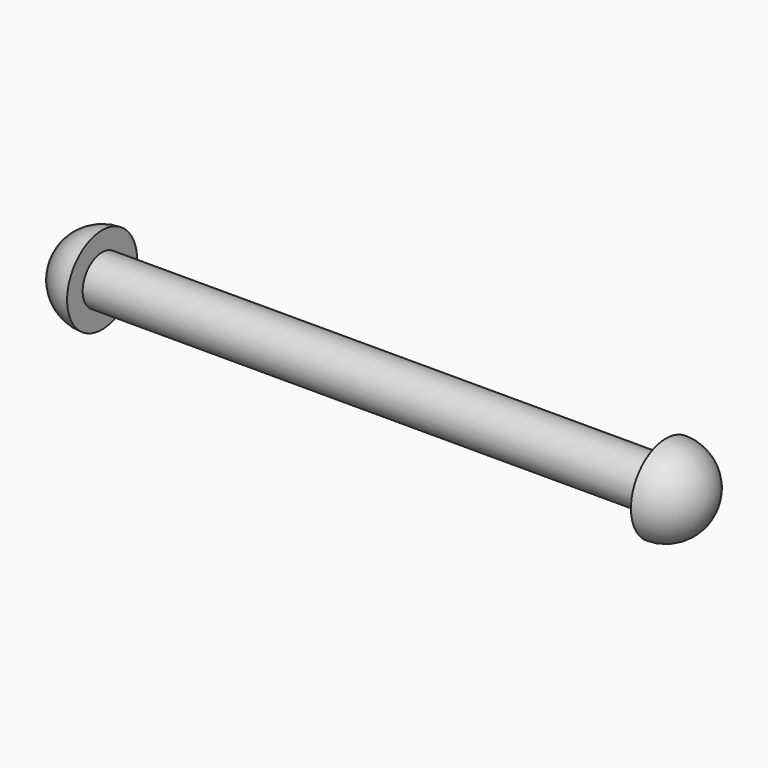
from build123d import *

# Parameters (mm, degrees)
F0_R     = 3.175
F1_DEPTH = 36.83


# Not quite as in the source:
# - a length typed as a fraction of an inch, garbled in the dataset ("3 / 203.2 mm" for 3/8 in), is restored
# - a feature names something its author has since deleted; it is built from what else it names


with BuildPart() as f1:
    # F0 (on Right) → F1 (new body)
    with BuildSketch(Plane.YZ):
        Circle(F0_R)
    extrude(amount=-F1_DEPTH)

    # F2 (on Front) → F3 (revolve)
    with BuildSketch(Plane.XZ):
        with BuildLine():
            Line((0, 3.175), (0, 0))
            Line((0, 0), (5.715, 0))
            ThreePointArc((5.715, 0), (4.0411152545, 4.0411152545), (0, 5.715))
            Line((0, 5.715), (0, 3.175))
        make_face()
    revolve(axis=Axis((0, 0, 0), (1, 0, 0)))

    # F4: F1 across face


with BuildPart() as f1_1:
    add(f1.part)
    add(f1.part.mirror(Plane(origin=(-36.83, 0, 0), x_dir=(0, 1, 0), z_dir=(-1, 0, 0))))


solid = f1_1.part
